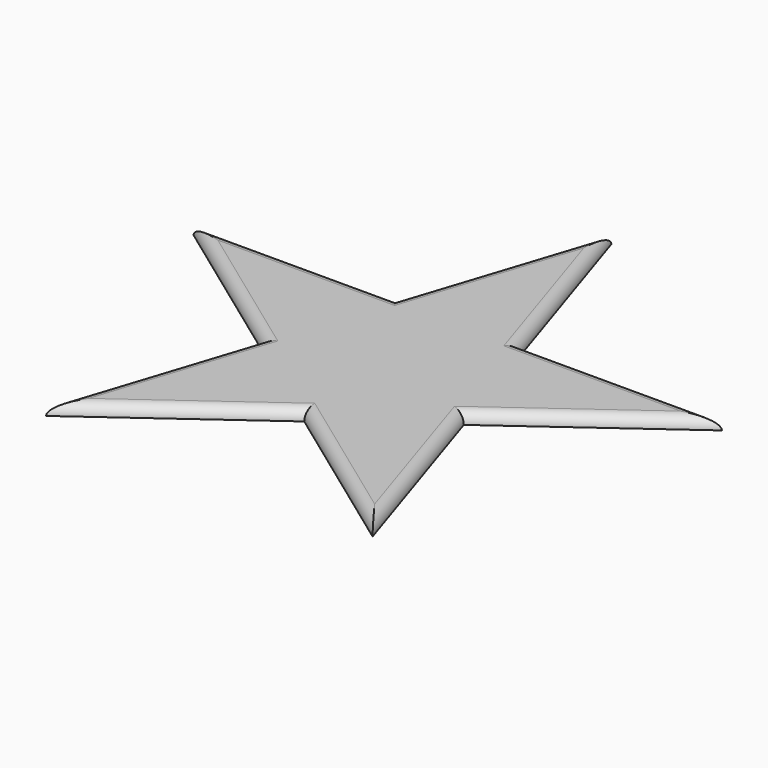
from build123d import *

# Parameters (mm, degrees)
F1_DEPTH = 2.5
F2_R     = 2.49999


# Not quite as in the source:
# - a fillet or chamfer is up to 0.001 mm smaller than in the source, because OpenCascade refuses the exact size


with BuildPart() as f1:
    # F0 (on Top) → F1 (new body)
    with BuildSketch(Plane.XY):
        Polygon((-14.5934092388, 20.0861046344), (-61.8186735592, 20.0861046344), (-23.6126321602, -7.6722092687), (-38.206041399, -52.5861046344), (0, -24.8277907313), (38.206041399, -52.5861046344), (23.6126321602, -7.6722092687), (61.8186735592, 20.0861046344), (14.5934092388, 20.0861046344), (0, 65), align=None)
    extrude(amount=F1_DEPTH)

    # F2 (radius 2.5 in the source; OpenCascade refuses exactly that, so slightly less here)
    f2_edges = [f1.edges().sort_by_distance(p)[0] for p in [
        (-7.296705, 42.543052, 2.5),
        (-38.206041, 20.086105, 2.5),
        (-42.715653, 6.206948, 2.5),
        (-30.909337, -30.129157, 2.5),
        (19.103021, -38.706948, 2.5),
        (30.909337, -30.129157, 2.5),
        (42.715653, 6.206948, 2.5),
        (38.206041, 20.086105, 2.5),
        (7.296705, 42.543052, 2.5),
        (-19.103021, -38.706948, 2.5),
    ]]
    fillet(f2_edges, radius=F2_R)


solid = f1.part
